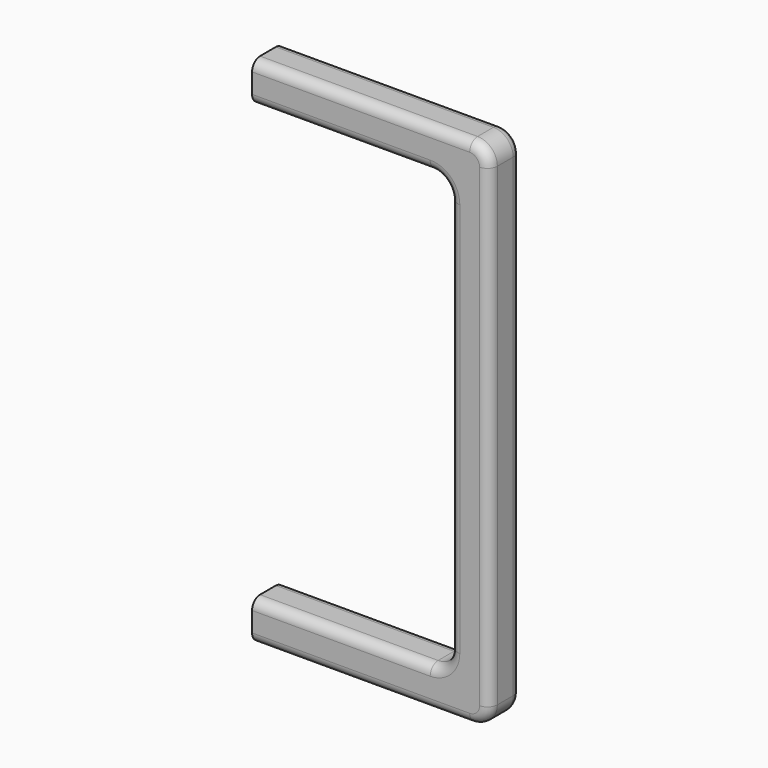
from build123d import *

# Parameters (mm, degrees)
F3_DEPTH = 3.175
F4_R     = 1.5875


# Not quite as in the source:
# - the program builds the solid bodies; features that only make, move or delete a surface that nothing else refers to are left out


with BuildPart() as f3:
    # F2 (on Front) → F3 (new body, symmetric)
    with BuildSketch(Plane.XZ):
        with BuildLine():
            Line((72.3697372794, 95.25), (37.3974703252, 95.25))
            Line((37.3974703252, 95.25), (37.3974703252, 88.9))
            Line((37.3974703252, 88.9), (66.0197372794, 88.9))
            ThreePointArc((66.0197372794, 88.9), (68.2648013097, 87.9700640303), (69.1947372794, 85.725))
            Line((69.1947372794, 85.725), (69.1947372794, 22.225))
            ThreePointArc((69.1947372794, 22.225), (68.2648013097, 19.9799359697), (66.0197372794, 19.05))
            Line((66.0197372794, 19.05), (37.3974703252, 19.05))
            Line((37.3974703252, 19.05), (37.3974703252, 12.7))
            Line((37.3974703252, 12.7), (72.3697372794, 12.7))
            ThreePointArc((72.3697372794, 12.7), (74.6148013097, 13.6299359697), (75.5447372794, 15.875))
            Line((75.5447372794, 15.875), (75.5447372794, 92.075))
            ThreePointArc((75.5447372794, 92.075), (74.6148013097, 94.3200640303), (72.3697372794, 95.25))
        make_face()
    extrude(amount=F3_DEPTH, both=True)

    # F4
    f4_edges = [f3.edges().sort_by_distance(p)[0] for p in [
        (54.883604, -3.175, 12.7),
        (54.883604, 3.175, 12.7),
        (51.708604, 3.175, 19.05),
        (51.708604, -3.175, 19.05),
    ]]
    fillet(f4_edges, radius=F4_R)


solid = f3.part
